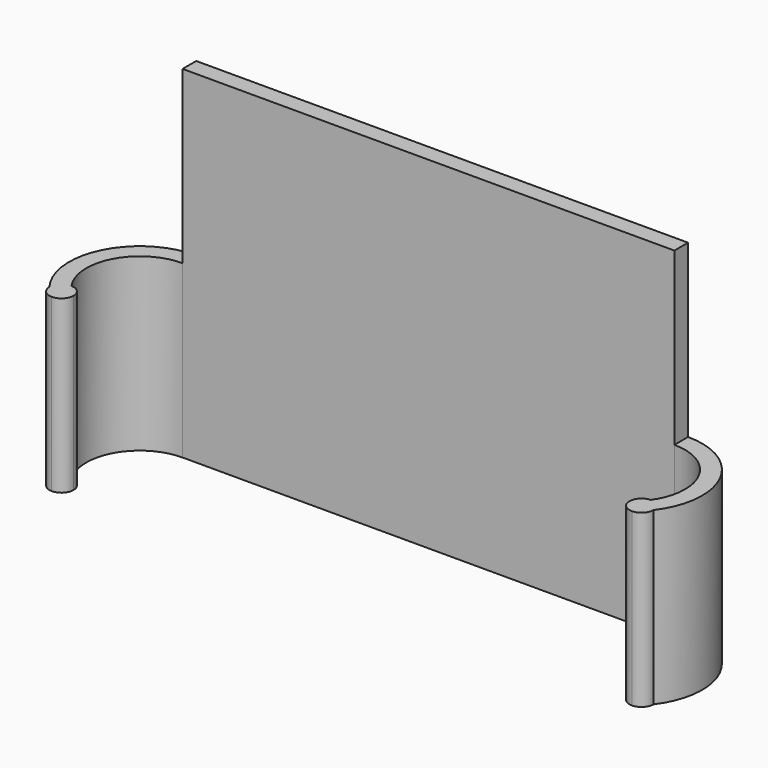
from build123d import *

# Parameters (mm, degrees)
F1_DEPTH = 20
F2_W     = 18.2070606947
F2_H     = 20
F2_W_2   = 57.5
F2_W_3   = 18.4121565521
F3_DEPTH = 25
F4_DEPTH = 25


# Not quite as in the source:
# - a pattern or mirror of a feature is missing from the dataset's text; its kind, count and spacing are read off the source's solid


with BuildPart() as f1:
    # F0 (on Top) → F1 (new body, symmetric)
    with BuildSketch(Plane.XY):
        with BuildLine():
            Line((-28.75, 8.25), (-28.75, 6.25))
            Line((-28.75, 6.25), (-23.3648351929, 6.25))
            ThreePointArc((-23.3648351929, 6.25), (-25.8777186767, 7.7338541491), (-28.75, 8.25))
        make_face()
        with BuildLine():
            ThreePointArc((-33.8628873162, -3.5945630182), (-34.2965538339, 2.8806666881), (-28.75, 6.25))
            Line((-28.75, 6.25), (-28.75, 8.25))
            ThreePointArc((-28.75, 8.25), (-36.1429865413, 3.661454629), (-35.3122023742, -5))
            ThreePointArc((-35.3122023742, -5), (-34.8849672334, -3.9905735233), (-33.8628873162, -3.5945630182))
        make_face()
        with BuildLine():
            ThreePointArc((-28.75, 8.25), (-25.8777186767, 7.7338541491), (-23.3648351929, 6.25))
            Line((-23.3648351929, 6.25), (23.3648351929, 6.25))
            ThreePointArc((23.3648351929, 6.25), (25.8777186767, 7.7338541491), (28.75, 8.25))
            Line((28.75, 8.25), (-28.75, 8.25))
        make_face()
        with BuildLine():
            ThreePointArc((-32.5, -5), (-32.8966747104, -4.0211339537), (-33.8628873162, -3.5945630182))
            ThreePointArc((-33.8628873162, -3.5945630182), (-33.2368147022, -4.3509761925), (-32.5, -5))
        make_face()
        with BuildLine():
            ThreePointArc((-32.5, -5), (-33.2368147022, -4.3509761925), (-33.8628873162, -3.5945630182))
            ThreePointArc((-33.8628873162, -3.5945630182), (-34.8849672334, -3.9905735233), (-35.3122023742, -5))
            Line((-35.3122023742, -5), (-32.5, -5))
        make_face()
        with BuildLine():
            ThreePointArc((28.75, 8.25), (25.8777186767, 7.7338541491), (23.3648351929, 6.25))
            Line((23.3648351929, 6.25), (28.75, 6.25))
            Line((28.75, 6.25), (28.75, 8.25))
        make_face()
        with BuildLine():
            ThreePointArc((-33.949315058, -6.4054369818), (-32.9272351408, -6.0094264767), (-32.5, -5))
            Line((-32.5, -5), (-35.3122023742, -5))
            ThreePointArc((-35.3122023742, -5), (-34.672595407, -5.7432885741), (-33.949315058, -6.4054369818))
        make_face()
        with BuildLine():
            ThreePointArc((-33.949315058, -6.4054369818), (-34.672595407, -5.7432885741), (-35.3122023742, -5))
            ThreePointArc((-35.3122023742, -5), (-34.9155276638, -5.9788660463), (-33.949315058, -6.4054369818))
        make_face()
    extrude(amount=F1_DEPTH, both=True)



with BuildPart() as f1b:
    # F0 (on Top) → F1, piece 2 (new body, symmetric)
    with BuildSketch(Plane.XY):
        with BuildLine():
            ThreePointArc((33.949315058, -6.4054369818), (34.9155276638, -5.9788660463), (35.3122023742, -5))
            ThreePointArc((35.3122023742, -5), (34.672595407, -5.7432885741), (33.949315058, -6.4054369818))
        make_face()
        with BuildLine():
            ThreePointArc((33.949315058, -6.4054369818), (34.672595407, -5.7432885741), (35.3122023742, -5))
            Line((35.3122023742, -5), (32.5, -5))
            ThreePointArc((32.5, -5), (32.9272351408, -6.0094264767), (33.949315058, -6.4054369818))
        make_face()
        with BuildLine():
            Line((32.5, -5), (35.3122023742, -5))
            ThreePointArc((35.3122023742, -5), (34.8849672334, -3.9905735233), (33.8628873162, -3.5945630182))
            ThreePointArc((33.8628873162, -3.5945630182), (33.2368147022, -4.3509761925), (32.5, -5))
        make_face()
    extrude(amount=F1_DEPTH, both=True)


with BuildPart() as f1_1:
    add(f1.part)

    add(f1b.part)  # F1_copies merges F1b
    # F1_copies: F1 across plane
    add(f1.part.mirror(Plane(origin=(0, 0, 0), x_dir=(0, 0, 1), z_dir=(1, 0, 0))))

    # F2 (on Front) → F3 (cut)
    with BuildSketch(Plane.XZ):
        with Locations((-37.8535303473, 10)):
            Rectangle(F2_W, F2_H)
        with Locations((0, 10)):
            Rectangle(F2_W_2, F2_H)
        with Locations((37.956078276, 10)):
            Rectangle(F2_W_3, F2_H)
    extrude(amount=F3_DEPTH, mode=Mode.SUBTRACT)

    # F2 (on Front) → F4 (cut)
    with BuildSketch(Plane.XZ):
        with Locations((-37.8535303473, 10)):
            Rectangle(F2_W, F2_H)
        with Locations((37.956078276, 10)):
            Rectangle(F2_W_3, F2_H)
    extrude(amount=-F4_DEPTH, mode=Mode.SUBTRACT)


solid = f1_1.part
